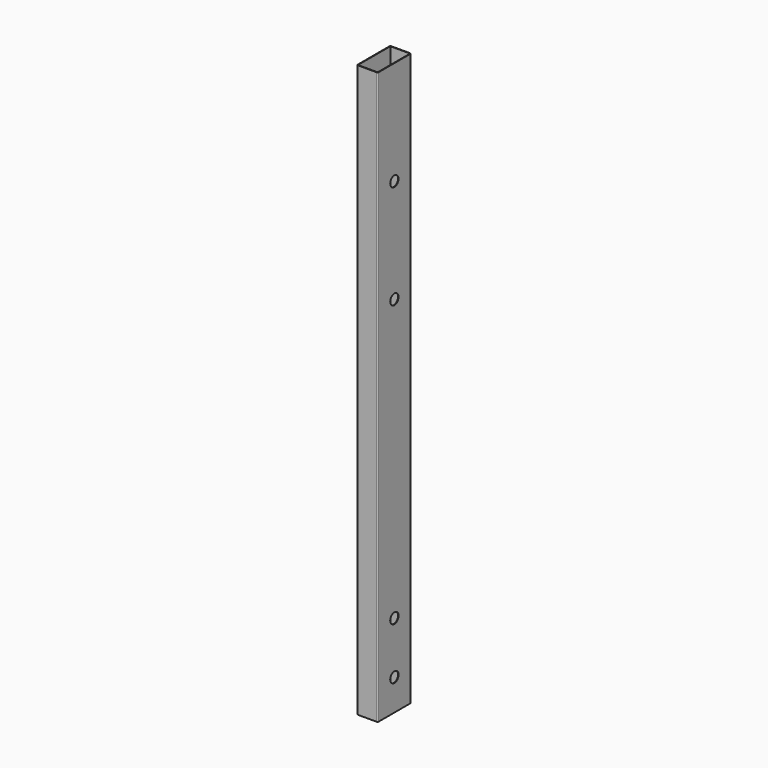
from build123d import *

# Parameters (mm, degrees)
F0_W     = 19
F0_H     = 39
F1_DEPTH = 550
F3_D     = 10
F3_DEPTH = 30
F3_TIP   = 3.0043030951


# Not quite as in the source:
# - a feature names something its author has since deleted; it is built from what else it names


with BuildPart() as f1:
    # F0 (on Top) → F1 (new body)
    with BuildSketch(Plane.XY):
        with BuildLine():
            Line((9, 20), (-9, 20))
            ThreePointArc((-9, 20), (-9.7071067812, 19.7071067812), (-10, 19))
            Line((-10, 19), (-10, -19))
            ThreePointArc((-10, -19), (-9.7071067812, -19.7071067812), (-9, -20))
            Line((-9, -20), (9, -20))
            ThreePointArc((9, -20), (9.7071067812, -19.7071067812), (10, -19))
            Line((10, -19), (10, 19))
            ThreePointArc((10, 19), (9.7071067812, 19.7071067812), (9, 20))
        make_face()
        Rectangle(F0_W, F0_H, mode=Mode.SUBTRACT)
    extrude(amount=F1_DEPTH)

    # F3
    with Locations(Plane.YZ.offset(10)):
        with Locations((0, 80), (0, 30), (0, 450), (0, 350)):
            Hole(F3_D / 2, depth=F3_DEPTH)
            with Locations((0, 0, -(F3_DEPTH + F3_TIP / 2))):  # 118° drill point
                Cone(0, F3_D / 2, F3_TIP, mode=Mode.SUBTRACT)


solid = f1.part
